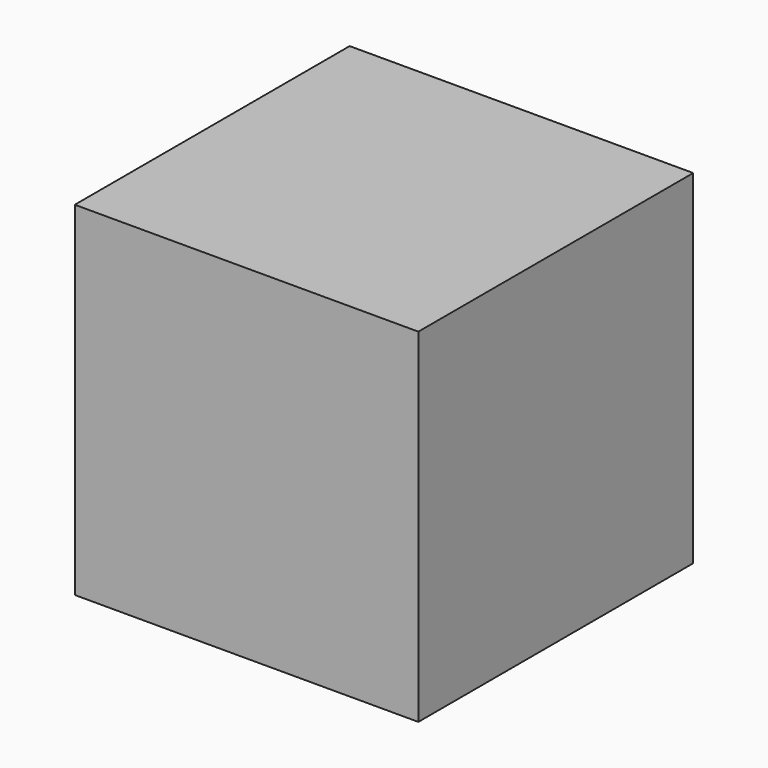
from build123d import *

# Parameters (mm, degrees)
F0_W     = 1000
F0_H     = 1000
F1_DEPTH = 1000


# Not quite as in the source:
# - a feature of the source that left no trace in its solid (it failed there, or was rolled back) is left out


with BuildPart() as f1:
    # F0 (on Front) → F1 (new body)
    with BuildSketch(Plane.XZ):
        with Locations((500, 500)):
            Rectangle(F0_W, F0_H)
    extrude(amount=-F1_DEPTH)


solid = f1.part
